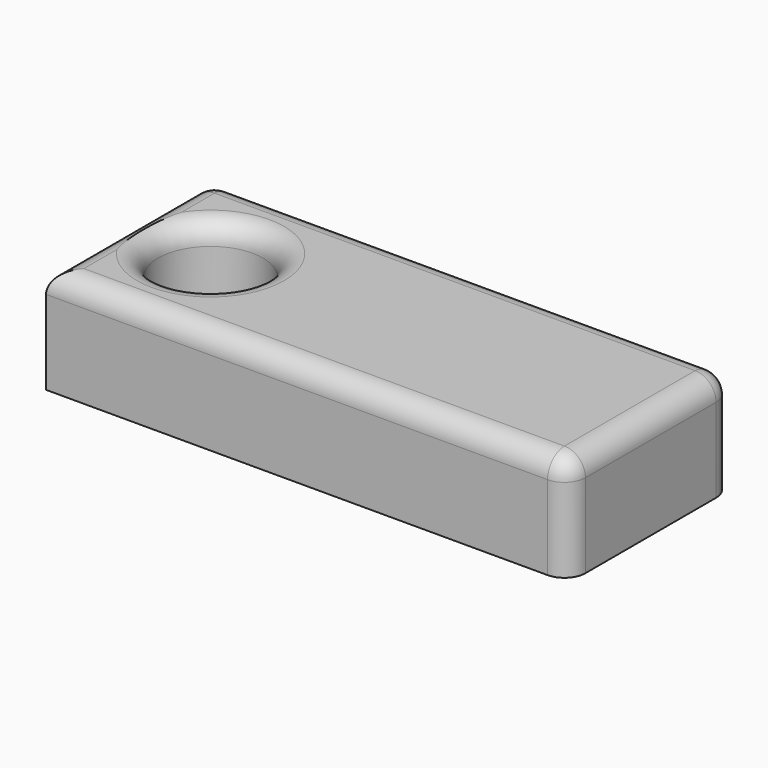
from build123d import *

# Parameters (mm, degrees)
F0_W         = 124.3421025574
F0_H         = 48.8486886024
F1_DEPTH     = 25
F3_D         = 25
F4_T1_DEPTH  = 149.3421025574
F4_T3_DEPTH  = 73.8486886024
F5_T1_DEPTH  = 32.5
F5_S5_W      = 5
F5_S5_H      = 5
F5_T6_DEPTH  = 5
F6_T1_DEPTH  = 32.5
F6_S5_W      = 5
F6_S5_H      = 5
F6_T6_DEPTH  = 5
F6_S11_W     = 5
F6_S11_H     = 5
F6_T12_DEPTH = 5


# Not quite as in the source:
# - a fillet or chamfer that OpenCascade refuses, or shapes differently, is made with other operations: its cross-section is extruded or revolved along the edge and cut away or added


with BuildPart() as f1:
    # F0 (on Top) → F1 (new body)
    with BuildSketch(Plane.XY):
        with Locations((-25.8323382586, 0)):
            Rectangle(F0_W, F0_H)
    extrude(amount=F1_DEPTH)

    # F3 (through all)
    with Locations(Plane.XY.offset(25)):
        with Locations((-68.3952495456, 0)):
            Hole(F3_D / 2)

    # F4: fillet of radius 5 on 5 edges, made by hand

    # F4_s2 → F4_t1 (cut)
    with BuildSketch(Plane.YZ.offset(-100.5033895373)):
        with BuildLine():
            ThreePointArc((24.4243443012, 20), (22.9598782072, 23.5355339059), (19.4243443012, 25))
            Line((19.4243443012, 25), (24.4243443012, 25))
            Line((24.4243443012, 25), (24.4243443012, 20))
        make_face()
        with BuildLine():
            ThreePointArc((-19.4243443012, 25), (-22.9598782072, 23.5355339059), (-24.4243443012, 20))
            Line((-24.4243443012, 20), (-24.4243443012, 25))
            Line((-24.4243443012, 25), (-19.4243443012, 25))
        make_face()
    extrude(amount=F4_T1_DEPTH, mode=Mode.SUBTRACT)

    # F4_s4 → F4_t3 (cut)
    with BuildSketch(Plane.XZ.offset(-36.9243443012)):
        with BuildLine():
            ThreePointArc((36.3387130201, 20), (34.874246926, 23.5355339059), (31.3387130201, 25))
            Line((31.3387130201, 25), (36.3387130201, 25))
            Line((36.3387130201, 25), (36.3387130201, 20))
        make_face()
        with BuildLine():
            ThreePointArc((-88.0033895373, 20), (-86.5389234433, 23.5355339059), (-83.0033895373, 25))
            Line((-83.0033895373, 25), (-88.0033895373, 25))
            Line((-88.0033895373, 25), (-88.0033895373, 20))
        make_face()
    extrude(amount=F4_T3_DEPTH, mode=Mode.SUBTRACT)

    # F4_s5 → F4_t6 (revolve, cut)
    with BuildSketch(Plane.XZ):
        with BuildLine():
            ThreePointArc((-50.8952495456, 25), (-54.4307834515, 23.5355339059), (-55.8952495456, 20))
            Line((-55.8952495456, 20), (-55.8952495456, 25))
            Line((-55.8952495456, 25), (-50.8952495456, 25))
        make_face()
    revolve(axis=Axis((-68.3952495456, 0, 25), (0, 0, 1)), mode=Mode.SUBTRACT)

    # F5: fillet of radius 5 on 1 edges, made by hand

    # F5_s2 → F5_t1 (cut)
    with BuildSketch(Plane.XY.offset(-12.5)):
        with BuildLine():
            ThreePointArc((36.3387130201, -19.4243443012), (34.874246926, -22.9598782072), (31.3387130201, -24.4243443012))
            Line((31.3387130201, -24.4243443012), (36.3387130201, -24.4243443012))
            Line((36.3387130201, -24.4243443012), (36.3387130201, -19.4243443012))
        make_face()
    extrude(amount=F5_T1_DEPTH, mode=Mode.SUBTRACT)


with BuildPart() as f5_tool4:
    # F5_s5 → F5_t6 (new body)
    with BuildSketch(Plane.YZ.offset(31.3387130201)):
        with Locations((-21.9243443012, 22.5)):
            Rectangle(F5_S5_W, F5_S5_H)
    extrude(amount=F5_T6_DEPTH)

    # F5_s7 → F5_t8 (revolve, cut)
    with BuildSketch(Plane(origin=(31.3387130201, -19.4243443012, 20), x_dir=(0, 0.7071067812, -0.7071067812), z_dir=(0, -0.7071067812, -0.7071067812))):
        with BuildLine():
            ThreePointArc((0, -5), (5, 0), (0, 5))
            Line((0, 5), (0, -5))
        make_face()
    revolve(axis=Axis((31.3387130201, -19.4243443012, 20), (1, 0, 0)), mode=Mode.SUBTRACT)


with BuildPart() as f1_1:
    add(f1.part)

    # F5_t3: cut F5_tool4
    add(f5_tool4.part, mode=Mode.SUBTRACT)

    # F6: fillet of radius 5 on 2 edges, made by hand

    # F6_s2 → F6_t1 (cut)
    with BuildSketch(Plane.XY.offset(-12.5)):
        with BuildLine():
            ThreePointArc((-83.0033895373, 24.4243443012), (-86.5389234433, 22.9598782072), (-88.0033895373, 19.4243443012))
            Line((-88.0033895373, 19.4243443012), (-88.0033895373, 24.4243443012))
            Line((-88.0033895373, 24.4243443012), (-83.0033895373, 24.4243443012))
        make_face()
        with BuildLine():
            ThreePointArc((31.3387130201, 24.4243443012), (34.874246926, 22.9598782072), (36.3387130201, 19.4243443012))
            Line((36.3387130201, 19.4243443012), (36.3387130201, 24.4243443012))
            Line((36.3387130201, 24.4243443012), (31.3387130201, 24.4243443012))
        make_face()
    extrude(amount=F6_T1_DEPTH, mode=Mode.SUBTRACT)


with BuildPart() as f6_tool4:
    # F6_s5 → F6_t6 (new body)
    with BuildSketch(Plane.XZ.offset(-19.4243443012)):
        with Locations((33.8387130201, 22.5)):
            Rectangle(F6_S5_W, F6_S5_H)
    extrude(amount=-F6_T6_DEPTH)

    # F6_s7 → F6_t8 (revolve, cut)
    with BuildSketch(Plane(origin=(31.3387130201, 19.4243443012, 20), x_dir=(-0.7071067812, 0, -0.7071067812), z_dir=(0.7071067812, 0, -0.7071067812))):
        with BuildLine():
            ThreePointArc((0, -5), (5, 0), (0, 5))
            Line((0, 5), (0, -5))
        make_face()
    revolve(axis=Axis((31.3387130201, 19.4243443012, 20), (0, 1, 0)), mode=Mode.SUBTRACT)


with BuildPart() as f1_2:
    add(f1_1.part)

    # F6_t3: cut F6_tool4
    add(f6_tool4.part, mode=Mode.SUBTRACT)


with BuildPart() as f6_tool10:
    # F6_s11 → F6_t12 (new body)
    with BuildSketch(Plane.XZ.offset(-19.4243443012)):
        with Locations((-85.5033895373, 22.5)):
            Rectangle(F6_S11_W, F6_S11_H)
    extrude(amount=-F6_T12_DEPTH)

    # F6_s13 → F6_t14 (revolve, cut)
    with BuildSketch(Plane(origin=(-83.0033895373, 19.4243443012, 20), x_dir=(0.7071067812, 0, -0.7071067812), z_dir=(0.7071067812, 0, 0.7071067812))):
        with BuildLine():
            ThreePointArc((0, -5), (5, 0), (0, 5))
            Line((0, 5), (0, -5))
        make_face()
    revolve(axis=Axis((-83.0033895373, 19.4243443012, 20), (0, 1, 0)), mode=Mode.SUBTRACT)


with BuildPart() as f1_3:
    add(f1_2.part)

    # F6_t9: cut F6_tool10
    add(f6_tool10.part, mode=Mode.SUBTRACT)


solid = f1_3.part
